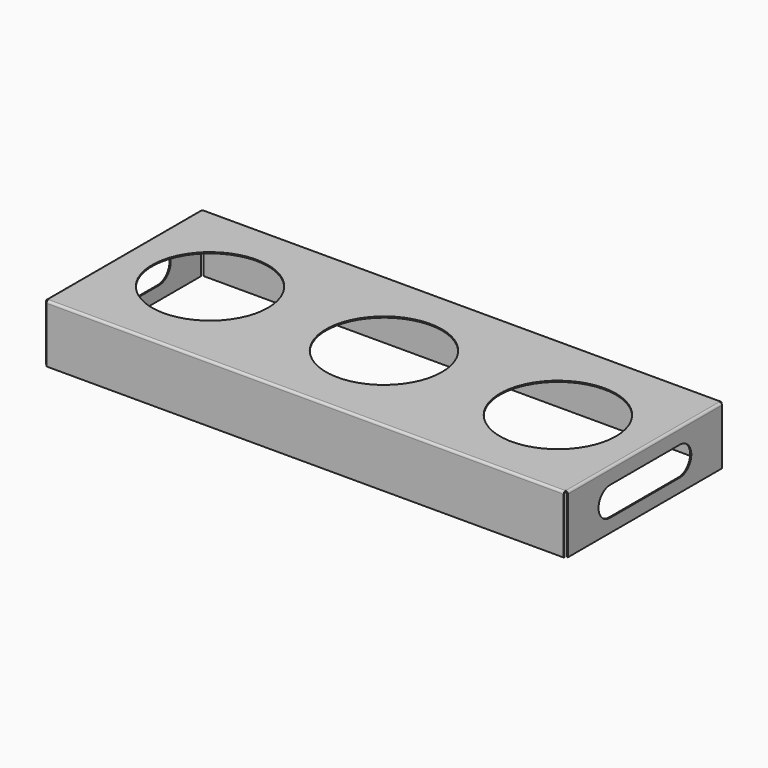
from build123d import *

# Parameters (mm, degrees)
F3_W           = 446
F3_H           = 166
F3_R           = 50
F4_DEPTH       = 1
F6_DEPTH       = 223
F8_DEPTH       = 83
F10_DEPTH      = 225.001
F10_DEPTH_BACK = 225.001


# Not quite as in the source:
# - a pattern or mirror of a feature is missing from the dataset's text; its kind, count and spacing are read off the source's solid


with BuildPart() as f4:
    # F3 (on Top) → F4 (new body)
    with BuildSketch(Plane.XY):
        Rectangle(F3_W, F3_H)
        with Locations((-150, 0)):
            Circle(F3_R, mode=Mode.SUBTRACT)
        Circle(F3_R, mode=Mode.SUBTRACT)
        with Locations((150, 0)):
            Circle(F3_R, mode=Mode.SUBTRACT)
    extrude(amount=F4_DEPTH)

    # F5 (on Right) → F6 (join, symmetric)
    with BuildSketch(Plane.YZ):
        with BuildLine():
            ThreePointArc((85, -1), (84.4142135624, 0.4142135624), (83, 1))
            Line((83, 1), (83, 0))
            ThreePointArc((83, 0), (83.7071067812, -0.2928932188), (84, -1))
            Line((84, -1), (84, -49))
            Line((84, -49), (85, -49))
            Line((85, -49), (85, -1))
        make_face()
    f6 = extrude(amount=F6_DEPTH, both=True)

    # F6_copies: F6 across plane
    add(f6.mirror(Plane(origin=(0, 0, 0), x_dir=(0, 0, -1), z_dir=(0, -1, 0))))

    # F7 (on Front) → F8 (join, symmetric)
    with BuildSketch(Plane.XZ):
        with BuildLine():
            ThreePointArc((225, -1), (224.4142135624, 0.4142135624), (223, 1))
            Line((223, 1), (223, 0))
            ThreePointArc((223, 0), (223.7071067812, -0.2928932188), (224, -1))
            Line((224, -1), (224, -49))
            Line((224, -49), (225, -49))
            Line((225, -49), (225, -1))
        make_face()
    f8 = extrude(amount=F8_DEPTH, both=True)

    # F8_copies: F8 across plane
    add(f8.mirror(Plane(origin=(0, 0, 0), x_dir=(0, 0, -1), z_dir=(-1, 0, 0))))

    # F9 (on Right) → F10 (cut, two sides)
    with BuildSketch(Plane.YZ) as f10_sk:
        with BuildLine():
            ThreePointArc((37.5, -37.5), (50, -25), (37.5, -12.5))
            Line((37.5, -12.5), (-37.5, -12.5))
            ThreePointArc((-37.5, -12.5), (-50, -25), (-37.5, -37.5))
            Line((-37.5, -37.5), (37.5, -37.5))
        make_face()
    extrude(amount=-F10_DEPTH, mode=Mode.SUBTRACT)
    extrude(f10_sk.sketch, amount=F10_DEPTH_BACK, mode=Mode.SUBTRACT)


solid = f4.part
